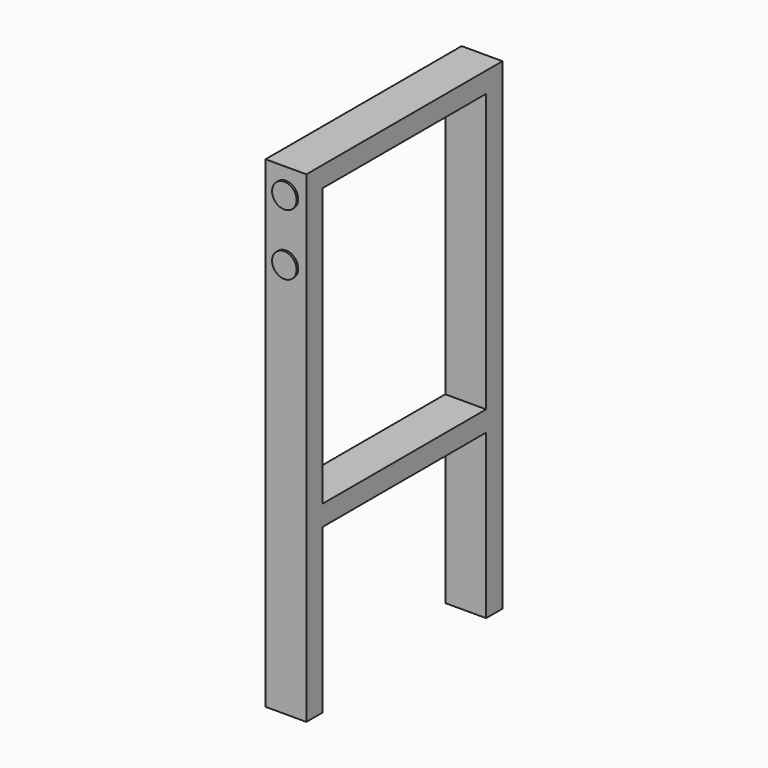
from build123d import *

# Parameters (mm, degrees)
F1_DEPTH = 12.7
F2_R     = 7.62
F3_DEPTH = 1.27


# Not quite as in the source:
# - a pattern or mirror of a feature is missing from the dataset's text; its kind, count and spacing are read off the source's solid


with BuildPart() as f1:
    # F0 (on Right) → F1 (new body, symmetric)
    with BuildSketch(Plane.YZ):
        Polygon((76.2, -149.86), (76.2, 149.86), (-76.2, 149.86), (-76.2, -149.86), (-63.5, -149.86), (-63.5, -48.26), (63.5, -48.26), (63.5, -149.86), align=None)
        Polygon((-63.5, 137.16), (0, 137.16), (63.5, 137.16), (63.5, -35.56), (-63.5, -35.56), align=None, mode=Mode.SUBTRACT)
    extrude(amount=F1_DEPTH, both=True)

    # F2 (on face) → F3 (join)
    with BuildSketch(Plane.XZ.offset(76.2)):
        with Locations((0, 96.52)):
            Circle(F2_R)
        with Locations((0, 134.62)):
            Circle(F2_R)
    f3 = extrude(amount=F3_DEPTH)

    # F3_copies: F3 across plane
    add(f3.mirror(Plane.ZX))


solid = f1.part
